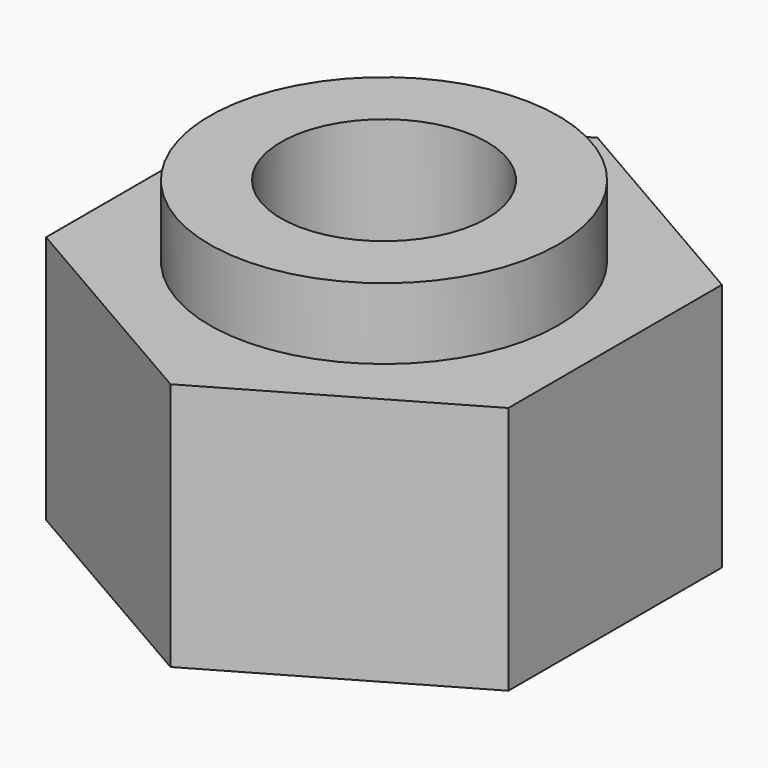
from build123d import *

# Parameters (mm, degrees)
F0_R     = 2.45
F0_R_2   = 1.45
F1_DEPTH = 2.5
F2_DEPTH = 2
F3_DEPTH = 3.5


# Not quite as in the source:
# - a feature names something its author has since deleted; it is built from what else it names


with BuildPart() as f1:
    # F0 (on Top) → F1 (new body)
    with BuildSketch(Plane.XY):
        Circle(F0_R)
        Circle(F0_R_2, mode=Mode.SUBTRACT)
    extrude(amount=F1_DEPTH)

    # F2 (add): a face of the model
    f2_faces = [f1.faces().sort_by_distance(p)[0] for p in [
        (-2.3807035354, 0, 2.5),
    ]]
    extrude(f2_faces, amount=F2_DEPTH)

    # F0 (on Top) → F3 (join)
    with BuildSketch(Plane.XY):
        Polygon((3.25, -1.8763883749), (3.25, 1.8763883749), (0, 3.7527767497), (-3.25, 1.8763883749), (-3.25, -1.8763883749), (0, -3.7527767497), align=None)
        Circle(F0_R, mode=Mode.SUBTRACT)
    extrude(amount=F3_DEPTH)


solid = f1.part
